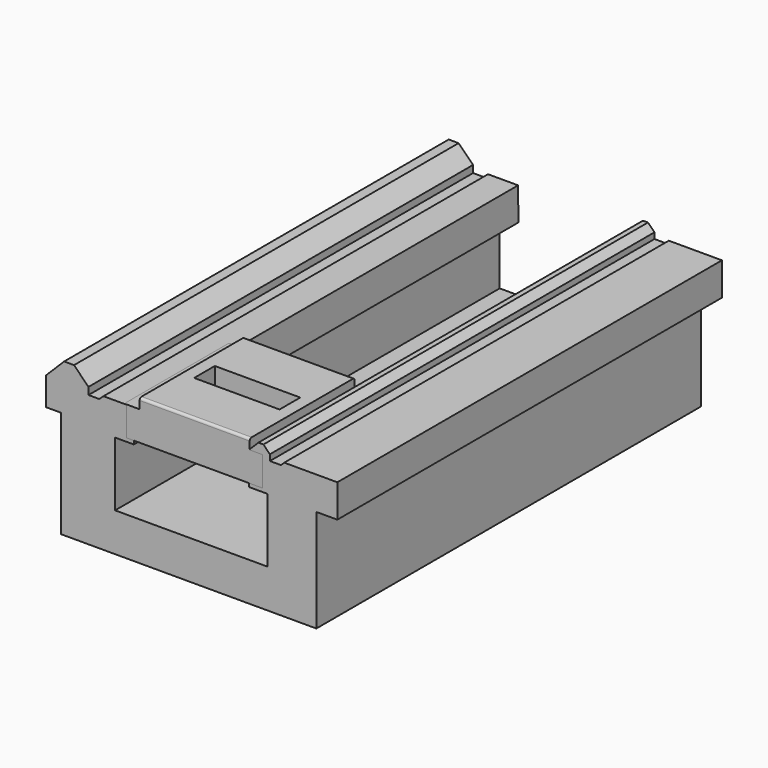
from build123d import *

# Parameters (mm, degrees)
F1_DEPTH     = 254
F3_DEPTH     = 69.342
F4_W         = 19.8628
F4_H         = 8.4582
F5_DEPTH     = 112.5890625953
F6_W         = 45.1358
F6_H         = 13.6652
F7_DEPTH     = 12.4714
F8_W         = 59.0677373111
F8_H         = 11.7043880746
F9_W         = 59.2527426779
F9_H         = 11.810824275
F10_DEPTH    = 12.7
F12_T1_DEPTH = 12.7
F12_2_F1_R   = 1.27
F12_2_F2_R   = 1.27
F12_2_F3_R   = 1.27


# Not quite as in the source:
# - a fillet or chamfer that OpenCascade refuses, or shapes differently, is made with other operations: its cross-section is extruded or revolved along the edge and cut away or added
# - a feature of the source that left no trace in its solid (it failed there, or was rolled back) is left out


with BuildPart() as f1:
    # F0 (on Front) → F1 (new body)
    with BuildSketch(Plane.XZ):
        Polygon((-32.1665374047, -17.3837374047), (-32.3189374047, -0.136982512), (-48.2193374047, -0.136982512), (-50.4037374047, -2.168982512), (-56.1187374047, -2.168982512), (-56.1187374047, 1.6204998967), (-63.759254996, 9.261017488), (-68.991654996, 9.261017488), (-78.5215374047, -0.2688649206), (-78.5215374047, -15.122982512), (-70.7375232514, -15.122982512), (-70.7375232514, -40.3150809519), (-70.7375232514, -51.727068197), (-70.7375232514, -71.6195074431), (64.27861262, -71.6195074431), (64.27861262, -51.727068197), (64.27861262, -37.3060261421), (64.27861262, -17.3837374047), (75.3770625953, -17.3837374047), (75.3770625953, -1.6865374047), (75.3770625953, 0.015417488), (73.5294523397, 0.015417488), (47.3022424863, 0.015417488), (45.6004424863, -1.686382512), (39.7408625953, -1.686382512), (39.7408625953, 1.4609331786), (36.3095782859, 4.892217488), (33.6594849986, 4.892217488), (28.6664625953, -0.1008049153), (28.6664625953, -17.3837374047), (38.5160344087, -17.3837374047), (38.5160344087, -19.4515101612), (38.5160344087, -51.2322857976), (-42.0471374047, -51.2322857976), (-42.0471374047, -17.3837374047), align=None)
    extrude(amount=-F1_DEPTH)


with BuildPart() as f3:
    # F2 (on Front) → F3 (new body)
    with BuildSketch(Plane.XZ):
        Polygon((-29.083, 0), (-37.211, 0), (-37.211, -15.5448), (37.211, -15.5448), (37.211, 0), (29.083, 0), (29.083, 5.3848), (-29.083, 5.3848), align=None)
    extrude(amount=-F3_DEPTH)

    # F4 (on face) → F5 (cut, through all)
    with BuildSketch(Plane(origin=(-37.211, 0, 0), x_dir=(0, -1, 0), z_dir=(-1, 0, 0))):
        with Locations((-34.671, -11.3157)):
            Rectangle(F4_W, F4_H)
    extrude(amount=-F5_DEPTH, mode=Mode.SUBTRACT)

    # F6 (on face) → F7 (cut, through all)
    with BuildSketch(Plane.XY.offset(5.3848)):
        with Locations((0, 34.671)):
            Rectangle(F6_W, F6_H)
    extrude(amount=-F7_DEPTH, mode=Mode.SUBTRACT)


with BuildPart() as f10_tool:
    # F8 (on face) + F9 (on face) → F10 (new body)
    with BuildSketch(Plane(origin=(0, 0, -15.5448), x_dir=(1, 0, 0), z_dir=(0, 0, -1))):
        with Locations((0, -14.4923576154)):
            Rectangle(F8_W, F8_H)
    with BuildSketch(Plane(origin=(0, 0, -15.5448), x_dir=(1, 0, 0), z_dir=(0, 0, -1))):
        with Locations((0.0775437802, -54.8617057502)):
            Rectangle(F9_W, F9_H)
    extrude(amount=-F10_DEPTH)


with BuildPart() as f1_1:
    add(f1.part)

    # F10: cut by f10_tool
    add(f10_tool.part, mode=Mode.SUBTRACT)

    # F12: fillet of radius 1.27 on 6 edges, made by hand

    # F12_s2 → F12_t1 (join)
    with BuildSketch(Plane.XY.offset(-15.5448)):
        with BuildLine():
            ThreePointArc((28.6664625953, 60.7671178877), (29.4107045782, 60.3302441705), (29.7039151192, 59.5185900861))
            Line((29.7039151192, 59.5185900861), (29.7039151192, 60.7671178877))
            Line((29.7039151192, 60.7671178877), (28.6664625953, 60.7671178877))
        make_face()
        with BuildLine():
            ThreePointArc((28.6664625953, 48.9562936127), (29.4107045782, 49.39316733), (29.7039151192, 50.2048214143))
            Line((29.7039151192, 50.2048214143), (29.7039151192, 48.9562936127))
            Line((29.7039151192, 48.9562936127), (28.6664625953, 48.9562936127))
        make_face()
        with BuildLine():
            ThreePointArc((28.6664625953, 8.6401635781), (29.2944496333, 9.1025017623), (29.5338686556, 9.8446626938))
            Line((29.5338686556, 9.8446626938), (29.5338686556, 8.6401635781))
            Line((29.5338686556, 8.6401635781), (28.6664625953, 8.6401635781))
        make_face()
        with BuildLine():
            ThreePointArc((28.6664625953, 20.3445516527), (29.2944496333, 19.8822134685), (29.5338686556, 19.140052537))
            Line((29.5338686556, 19.140052537), (29.5338686556, 20.3445516527))
            Line((29.5338686556, 20.3445516527), (28.6664625953, 20.3445516527))
        make_face()
    extrude(amount=F12_T1_DEPTH)


with BuildPart() as f3_1:
    add(f3.part)

    # F10: cut by f10_tool
    add(f10_tool.part, mode=Mode.SUBTRACT)

    # F12#2: fillet of radius 1.27 on 24 edges, made by hand

    # F12_2_f1
    f12_2_f1_edges = [f3_1.edges().sort_by_distance(p)[0] for p in [
        (29.7039151192, 60.7671178877, -9.1948),
        (29.7039151192, 48.9562936127, -9.1948),
        (29.5338686556, 8.6401635781, -9.1948),
        (29.5338686556, 20.3445516527, -9.1948),
        (-29.5338686556, 8.6401635781, -9.1948),
        (-29.5338686556, 20.3445516527, -9.1948),
        (-29.5488275588, 48.9562936127, -9.1948),
        (-29.5488275588, 60.7671178877, -9.1948),
    ]]
    fillet(f12_2_f1_edges, radius=F12_2_F1_R)

    # F12_2_f2
    f12_2_f2_edges = [f3_1.edges().sort_by_distance(p)[0] for p in [
        (37.211, 69.342, -7.7724),
        (-37.211, 69.342, -7.7724),
        (37.211, 0, -7.7724),
        (-37.211, 0, -7.7724),
        (0, 0, 5.3848),
        (0, 69.342, 5.3848),
        (-37.211, 56.9722, -15.5448),
        (-37.211, 12.3698, -15.5448),
        (37.211, 12.3698, -15.5448),
        (37.211, 56.9722, -15.5448),
    ]]
    fillet(f12_2_f2_edges, radius=F12_2_F2_R)

    # F12_2_f3
    f12_2_f3_edges = [f3_1.edges().sort_by_distance(p)[0] for p in [
        (0, 20.3445516527, -15.5448),
        (0.0775437802, 60.7671178877, -15.5448),
        (0, 8.6401635781, -15.5448),
        (-29.5338686556, 14.4923576154, -15.5448),
        (-29.5488275588, 54.8617057502, -15.5448),
        (0.0775437802, 48.9562936127, -15.5448),
        (29.3319407313, 49.3282680006, -15.5448),
        (-29.1768531709, 49.3282680006, -15.5448),
        (-29.1768531709, 60.3951434998, -15.5448),
        (-29.1618942677, 9.012137966, -15.5448),
        (-29.1618942677, 19.9725772648, -15.5448),
        (29.1618942677, 9.012137966, -15.5448),
        (29.3319407313, 60.3951434998, -15.5448),
        (29.1618942677, 19.9725772648, -15.5448),
    ]]
    fillet(f12_2_f3_edges, radius=F12_2_F3_R)


solid = Compound([f1_1.part, f3_1.part])
